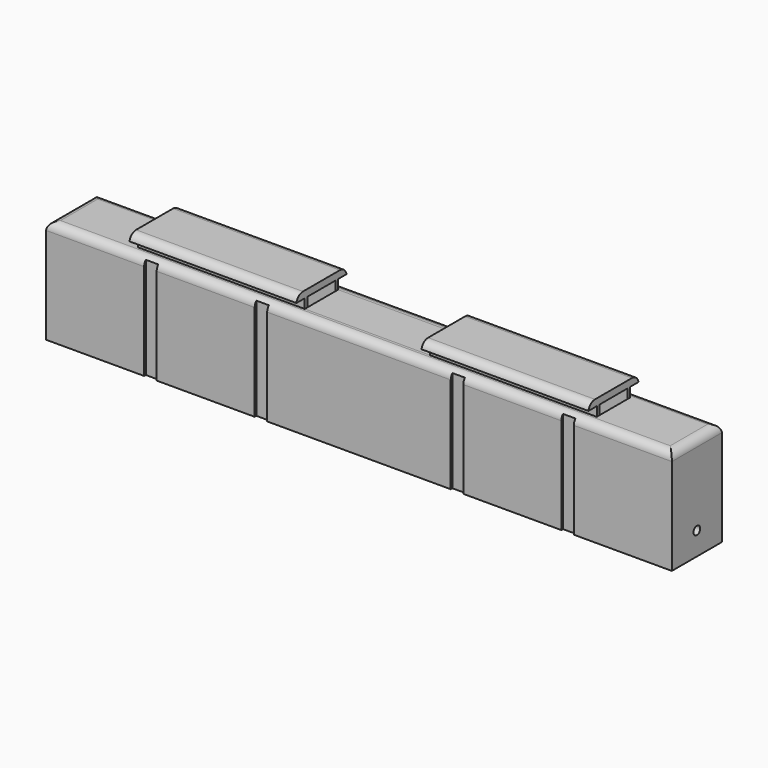
from build123d import *

# Parameters (mm, degrees)
F0_W           = 10.16
F0_H           = 2.54
F1_DEPTH       = 6.35
F2_DEPTH       = 0.635
F4_DEPTH       = 27.94
F6_R           = 0.254
F7_DEPTH       = 38.101
F8_T1_DEPTH    = 6.354829213
F8_T3_DEPTH    = 13.720829213
F10_DEPTH      = 9.652
F11_DEPTH      = 17.272
F12_W          = 2.5144716492
F12_H          = 3.5254987888
F13_DEPTH      = 3.81
F14_DEPTH      = 3.302
F16_DEPTH      = 10.16
F18_DEPTH      = 10.16
F20_DEPTH      = 10.16
F21_T1_DEPTH   = 12.6606557729
F23_DEPTH      = 10.16
F24_T1_DEPTH   = 12.6606557729
F24_2_T1_DEPTH = 8.0250460087
F24_2_T3_DEPTH = 8.0034146065
F24_2_T5_DEPTH = 8.0034146065
F24_2_T7_DEPTH = 8.0250460087
F25_W          = 7.62
F25_H          = 2.54
F26_DEPTH      = 4.5568268582
F27_W          = 7.62
F27_H          = 2.54
F28_DEPTH      = 4.5568268582


# Not quite as in the source:
# - a fillet or chamfer that OpenCascade refuses, or shapes differently, is made with other operations: its cross-section is extruded or revolved along the edge and cut away or added


with BuildPart() as f1:
    # F0 (on Top) → F1 (new body)
    with BuildSketch(Plane.XY):
        Polygon((13.081, -1.905), (19.05, -1.905), (19.05, 1.905), (13.081, 1.905), (13.081, 1.778), (12.319, 1.778), (12.319, 1.905), (6.35, 1.905), (6.35, 1.778), (5.588, 1.778), (5.588, 1.905), (-5.588, 1.905), (-5.588, 1.778), (-6.35, 1.778), (-6.35, 1.905), (-12.319, 1.905), (-12.319, 1.778), (-13.081, 1.778), (-13.081, 1.905), (-19.05, 1.905), (-19.05, -1.905), (-13.081, -1.905), (-13.081, -1.778), (-12.319, -1.778), (-12.319, -1.905), (-6.35, -1.905), (-6.35, -1.778), (-5.588, -1.778), (-5.588, -1.905), (5.588, -1.905), (5.588, -1.778), (6.35, -1.778), (6.35, -1.905), (12.319, -1.905), (12.319, -1.778), (13.081, -1.778), align=None)
        with Locations((-8.89, 0)):
            Rectangle(F0_W, F0_H, mode=Mode.SUBTRACT)
        with Locations((8.89, 0)):
            Rectangle(F0_W, F0_H, mode=Mode.SUBTRACT)
    extrude(amount=F1_DEPTH)

    # F0 (on Top) → F2 (join)
    with BuildSketch(Plane.XY):
        with Locations((-8.89, 0)):
            Rectangle(F0_W, F0_H)
        with Locations((8.89, 0)):
            Rectangle(F0_W, F0_H)
    extrude(amount=F2_DEPTH)

    # F3 (on face) → F4 (cut, through all)
    with BuildSketch(Plane.YZ.offset(-13.97)):
        Polygon((-0.4982374667, 0.381), (0.4982374667, 0.381), (0.4982374667, 0.889), (1.27, 1.397), (1.27, 5.461), (-1.27, 5.461), (-1.27, 1.397), (-0.4982374667, 0.889), align=None)
    extrude(amount=F4_DEPTH, mode=Mode.SUBTRACT)

    # F6 (on face) → F7 (cut, through all)
    with BuildSketch(Plane(origin=(-19.05, 0, 0), x_dir=(0, -1, 0), z_dir=(-1, 0, 0))):
        with Locations((0, 1.397)):
            Circle(F6_R)
    extrude(amount=-F7_DEPTH, mode=Mode.SUBTRACT)

    # F8: fillet of radius 0.508 on 4 edges, made by hand

    # F8_s2 → F8_t1 (cut)
    with BuildSketch(Plane.XZ.offset(-3.1774146065)):
        with BuildLine():
            ThreePointArc((-18.5410343146, 6.3504), (-18.9012102448, 6.2012102448), (-19.0504, 5.8410343146))
            Line((-19.0504, 5.8410343146), (-19.1013365685, 5.8410343146))
            ThreePointArc((-19.1013365685, 5.8410343146), (-19.1009365685, 6.0955171573), (-19.1009365685, 6.35))
            Line((-19.1009365685, 6.35), (-19.05, 6.4009365685))
            ThreePointArc((-19.05, 6.4009365685), (-18.7955171573, 6.4009365685), (-18.5410343146, 6.4013365685))
            Line((-18.5410343146, 6.4013365685), (-18.5410343146, 6.3504))
        make_face()
        with BuildLine():
            ThreePointArc((19.0504, 5.8410343146), (18.9012102448, 6.2012102448), (18.5410343146, 6.3504))
            Line((18.5410343146, 6.3504), (18.5410343146, 6.4013365685))
            ThreePointArc((18.5410343146, 6.4013365685), (18.7955171573, 6.4009365685), (19.05, 6.4009365685))
            Line((19.05, 6.4009365685), (19.1009365685, 6.35))
            ThreePointArc((19.1009365685, 6.35), (19.1009365685, 6.0955171573), (19.1013365685, 5.8410343146))
            Line((19.1013365685, 5.8410343146), (19.0504, 5.8410343146))
        make_face()
    extrude(amount=F8_T1_DEPTH, mode=Mode.SUBTRACT)

    # F8_s4 → F8_t3 (cut)
    with BuildSketch(Plane.YZ.offset(-6.8604146065)):
        with BuildLine():
            ThreePointArc((1.3960343146, 6.3504), (1.7562102448, 6.2012102448), (1.9054, 5.8410343146))
            Line((1.9054, 5.8410343146), (1.9563365685, 5.8410343146))
            ThreePointArc((1.9563365685, 5.8410343146), (1.9559365685, 6.0955171573), (1.9559365685, 6.35))
            Line((1.9559365685, 6.35), (1.905, 6.4009365685))
            ThreePointArc((1.905, 6.4009365685), (1.6505171573, 6.4009365685), (1.3960343146, 6.4013365685))
            Line((1.3960343146, 6.4013365685), (1.3960343146, 6.3504))
        make_face()
        with BuildLine():
            ThreePointArc((-1.3960343146, 6.3504), (-1.7562102448, 6.2012102448), (-1.9054, 5.8410343146))
            Line((-1.9054, 5.8410343146), (-1.9563365685, 5.8410343146))
            ThreePointArc((-1.9563365685, 5.8410343146), (-1.9559365685, 6.0955171573), (-1.9559365685, 6.35))
            Line((-1.9559365685, 6.35), (-1.905, 6.4009365685))
            ThreePointArc((-1.905, 6.4009365685), (-1.6505171573, 6.4009365685), (-1.3960343146, 6.4013365685))
            Line((-1.3960343146, 6.4013365685), (-1.3960343146, 6.3504))
        make_face()
    extrude(amount=F8_T3_DEPTH, mode=Mode.SUBTRACT)


with BuildPart() as f10:
    # F9 (on face) → F10 (new body, through all)
    with BuildSketch(Plane(origin=(-3.81, 0, 0), x_dir=(0, -1, 0), z_dir=(-1, 0, 0))):
        with BuildLine():
            Line((-0.0880359173, 1.4812426976), (-0.381, 5.207))
            ThreePointArc((-0.381, 5.207), (-0.9198153673, 4.9838153673), (-1.143, 4.445))
            Line((-1.143, 4.445), (-1.143, 1.397))
            Line((-1.143, 1.397), (-0.4176268994, 0.8964751032))
            ThreePointArc((-0.4176268994, 0.8964751032), (0, 0.4231398893), (0.4176268994, 0.8964751032))
            Line((0.4176268994, 0.8964751032), (1.143, 1.397))
            Line((1.143, 1.397), (1.143, 4.445))
            ThreePointArc((1.143, 4.445), (0.9198153673, 4.9838153673), (0.381, 5.207))
            Line((0.381, 5.207), (0.0880359173, 1.4812426976))
            ThreePointArc((0.0880359173, 1.4812426976), (0.1267060772, 1.4088201678), (0.0771916931, 1.3433317729))
            Line((0.0771916931, 1.3433317729), (0.0768500527, 1.338986977))
            Line((0.0768500527, 1.338986977), (0.0526172437, 1.0308073381))
            ThreePointArc((0.0526172437, 1.0308073381), (0, 0.6500122176), (-0.0526172437, 1.0308073381))
            Line((-0.0526172437, 1.0308073381), (-0.0768500527, 1.338986977))
            Line((-0.0768500527, 1.338986977), (-0.0771916931, 1.3433317729))
            ThreePointArc((-0.0771916931, 1.3433317729), (-0.1904525618, 1.4038076485), (-0.0880359173, 1.4812426976))
        make_face()
    extrude(amount=F10_DEPTH)

    # F11 (add, through all): a face of the model
    f11_faces = [f10.faces().sort_by_distance(p)[0] for p in [
        (-3.81, 0, 0.5969923029),
    ]]
    extrude(f11_faces, amount=F11_DEPTH)

    # F12 (on Right) → F13 (cut, symmetric)
    with BuildSketch(Plane.YZ):
        with Locations((-0.0007677008, 3.5559225362)):
            Rectangle(F12_W, F12_H)
    extrude(amount=F13_DEPTH, both=True, mode=Mode.SUBTRACT)


with BuildPart() as f14:
    # F14 (new): a face of the model
    f14_faces = [f1.part.faces().sort_by_distance(p)[0] for p in [
        (0, 0, 5.461),
    ]]
    extrude(f14_faces, amount=F14_DEPTH)

    # F27 (on face) → F28 (join, through all)
    with BuildSketch(Plane.XY.offset(1.7931731418)):
        Rectangle(F27_W, F27_H)
    extrude(amount=F28_DEPTH)


with BuildPart() as f1_1:
    add(f1.part)

    # F15 (on face) → F16 (cut, through all)
    with BuildSketch(Plane.YZ.offset(-13.97)):
        with BuildLine():
            Line((1.27, 4.572), (1.27, 4.318))
            ThreePointArc((1.27, 4.318), (1.397, 4.445), (1.27, 4.572))
        make_face()
        with BuildLine():
            ThreePointArc((-1.27, 4.572), (-1.397, 4.445), (-1.27, 4.318))
            Line((-1.27, 4.318), (-1.27, 4.572))
        make_face()
        with BuildLine():
            Line((-1.27, 4.953), (-1.27, 5.207))
            ThreePointArc((-1.27, 5.207), (-1.397, 5.08), (-1.27, 4.953))
        make_face()
        with BuildLine():
            ThreePointArc((1.27, 4.953), (1.397, 5.08), (1.27, 5.207))
            Line((1.27, 5.207), (1.27, 4.953))
        make_face()
    extrude(amount=F16_DEPTH, mode=Mode.SUBTRACT)

    # F17 (on face) → F18 (cut, through all)
    with BuildSketch(Plane(origin=(13.97, 0, 0), x_dir=(0, -1, 0), z_dir=(-1, 0, 0))):
        with BuildLine():
            Line((1.27, 4.5734065802), (1.27, 4.3194065802))
            ThreePointArc((1.27, 4.3194065802), (1.397, 4.4464065802), (1.27, 4.5734065802))
        make_face()
        with BuildLine():
            ThreePointArc((-1.27, 4.5734065802), (-1.397, 4.4464065802), (-1.27, 4.3194065802))
            Line((-1.27, 4.3194065802), (-1.27, 4.5734065802))
        make_face()
        with BuildLine():
            Line((-1.27, 4.9544065802), (-1.27, 5.2084065802))
            ThreePointArc((-1.27, 5.2084065802), (-1.397, 5.0814065802), (-1.27, 4.9544065802))
        make_face()
        with BuildLine():
            ThreePointArc((1.27, 4.9544065802), (1.397, 5.0814065802), (1.27, 5.2084065802))
            Line((1.27, 5.2084065802), (1.27, 4.9544065802))
        make_face()
    extrude(amount=F18_DEPTH, mode=Mode.SUBTRACT)

    # F24#2: fillet of radius 0.508 on 8 edges, made by hand

    # F24_2_s2 → F24_2_t1 (cut)
    with BuildSketch(Plane.YZ.offset(11.8085853935)):
        with BuildLine():
            ThreePointArc((-1.9054, 5.8410343146), (-1.7562102448, 6.2012102448), (-1.3960343146, 6.3504))
            Line((-1.3960343146, 6.3504), (-1.3960343146, 6.4013365685))
            ThreePointArc((-1.3960343146, 6.4013365685), (-1.6505171573, 6.4009365685), (-1.905, 6.4009365685))
            Line((-1.905, 6.4009365685), (-1.9559365685, 6.35))
            ThreePointArc((-1.9559365685, 6.35), (-1.9559365685, 6.0955171573), (-1.9563365685, 5.8410343146))
            Line((-1.9563365685, 5.8410343146), (-1.9054, 5.8410343146))
        make_face()
        with BuildLine():
            ThreePointArc((1.3960343146, 6.3504), (1.7562102448, 6.2012102448), (1.9054, 5.8410343146))
            Line((1.9054, 5.8410343146), (1.9563365685, 5.8410343146))
            ThreePointArc((1.9563365685, 5.8410343146), (1.9559365685, 6.0955171573), (1.9559365685, 6.35))
            Line((1.9559365685, 6.35), (1.905, 6.4009365685))
            ThreePointArc((1.905, 6.4009365685), (1.6505171573, 6.4009365685), (1.3960343146, 6.4013365685))
            Line((1.3960343146, 6.4013365685), (1.3960343146, 6.3504))
        make_face()
    extrude(amount=F24_2_T1_DEPTH, mode=Mode.SUBTRACT)

    # F24_2_s4 → F24_2_t3 (cut)
    with BuildSketch(Plane.YZ.offset(5.588)):
        with BuildLine():
            ThreePointArc((-1.3960343146, 6.3504), (-1.7562102448, 6.2012102448), (-1.9054, 5.8410343146))
            Line((-1.9054, 5.8410343146), (-1.9563365685, 5.8410343146))
            ThreePointArc((-1.9563365685, 5.8410343146), (-1.9559365685, 6.0955171573), (-1.9559365685, 6.35))
            Line((-1.9559365685, 6.35), (-1.905, 6.4009365685))
            ThreePointArc((-1.905, 6.4009365685), (-1.6505171573, 6.4009365685), (-1.3960343146, 6.4013365685))
            Line((-1.3960343146, 6.4013365685), (-1.3960343146, 6.3504))
        make_face()
        with BuildLine():
            ThreePointArc((1.3960343146, 6.3504), (1.7562102448, 6.2012102448), (1.9054, 5.8410343146))
            Line((1.9054, 5.8410343146), (1.9563365685, 5.8410343146))
            ThreePointArc((1.9563365685, 5.8410343146), (1.9559365685, 6.0955171573), (1.9559365685, 6.35))
            Line((1.9559365685, 6.35), (1.905, 6.4009365685))
            ThreePointArc((1.905, 6.4009365685), (1.6505171573, 6.4009365685), (1.3960343146, 6.4013365685))
            Line((1.3960343146, 6.4013365685), (1.3960343146, 6.3504))
        make_face()
    extrude(amount=F24_2_T3_DEPTH, mode=Mode.SUBTRACT)

    # F24_2_s6 → F24_2_t5 (cut)
    with BuildSketch(Plane.YZ.offset(-13.5914146065)):
        with BuildLine():
            ThreePointArc((-1.3960343146, 6.3504), (-1.7562102448, 6.2012102448), (-1.9054, 5.8410343146))
            Line((-1.9054, 5.8410343146), (-1.9563365685, 5.8410343146))
            ThreePointArc((-1.9563365685, 5.8410343146), (-1.9559365685, 6.0955171573), (-1.9559365685, 6.35))
            Line((-1.9559365685, 6.35), (-1.905, 6.4009365685))
            ThreePointArc((-1.905, 6.4009365685), (-1.6505171573, 6.4009365685), (-1.3960343146, 6.4013365685))
            Line((-1.3960343146, 6.4013365685), (-1.3960343146, 6.3504))
        make_face()
        with BuildLine():
            ThreePointArc((1.3960343146, 6.3504), (1.7562102448, 6.2012102448), (1.9054, 5.8410343146))
            Line((1.9054, 5.8410343146), (1.9563365685, 5.8410343146))
            ThreePointArc((1.9563365685, 5.8410343146), (1.9559365685, 6.0955171573), (1.9559365685, 6.35))
            Line((1.9559365685, 6.35), (1.905, 6.4009365685))
            ThreePointArc((1.905, 6.4009365685), (1.6505171573, 6.4009365685), (1.3960343146, 6.4013365685))
            Line((1.3960343146, 6.4013365685), (1.3960343146, 6.3504))
        make_face()
    extrude(amount=F24_2_T5_DEPTH, mode=Mode.SUBTRACT)

    # F24_2_s8 → F24_2_t7 (cut)
    with BuildSketch(Plane.YZ.offset(-19.8336314022)):
        with BuildLine():
            ThreePointArc((-1.3960343146, 6.3504), (-1.7562102448, 6.2012102448), (-1.9054, 5.8410343146))
            Line((-1.9054, 5.8410343146), (-1.9563365685, 5.8410343146))
            ThreePointArc((-1.9563365685, 5.8410343146), (-1.9559365685, 6.0955171573), (-1.9559365685, 6.35))
            Line((-1.9559365685, 6.35), (-1.905, 6.4009365685))
            ThreePointArc((-1.905, 6.4009365685), (-1.6505171573, 6.4009365685), (-1.3960343146, 6.4013365685))
            Line((-1.3960343146, 6.4013365685), (-1.3960343146, 6.3504))
        make_face()
        with BuildLine():
            ThreePointArc((1.3960343146, 6.3504), (1.7562102448, 6.2012102448), (1.9054, 5.8410343146))
            Line((1.9054, 5.8410343146), (1.9563365685, 5.8410343146))
            ThreePointArc((1.9563365685, 5.8410343146), (1.9559365685, 6.0955171573), (1.9559365685, 6.35))
            Line((1.9559365685, 6.35), (1.905, 6.4009365685))
            ThreePointArc((1.905, 6.4009365685), (1.6505171573, 6.4009365685), (1.3960343146, 6.4013365685))
            Line((1.3960343146, 6.4013365685), (1.3960343146, 6.3504))
        make_face()
    extrude(amount=F24_2_T7_DEPTH, mode=Mode.SUBTRACT)

    # F25 (on face) → F26 (cut, through all)
    with BuildSketch(Plane.XY.offset(6.35)):
        Rectangle(F25_W, F25_H)
    extrude(amount=-F26_DEPTH, mode=Mode.SUBTRACT)


with BuildPart() as f20:
    # F19 (on face) → F20 (new body, through all)
    with BuildSketch(Plane(origin=(13.97, 0, 0), x_dir=(0, -1, 0), z_dir=(-1, 0, 0))):
        with BuildLine():
            Line((-1.27, 4.9036065802), (-1.27, 3.7397078704))
            Line((-1.27, 3.7397078704), (-1.0667999741, 3.7397078704))
            Line((-1.0667999741, 3.7397078704), (-1.0667999741, 3.9429078963))
            Line((-1.0667999741, 3.9429078963), (-1.0667999741, 6.9219944999))
            Line((-1.0667999741, 6.9219944999), (1.0667999741, 6.9219944999))
            Line((1.0667999741, 6.9219944999), (1.0667999741, 4.4092186605))
            Line((1.0667999741, 4.4092186605), (1.0667999741, 3.7397078704))
            Line((1.0667999741, 3.7397078704), (1.27, 3.7397078704))
            Line((1.27, 3.7397078704), (1.27, 4.9036065802))
            ThreePointArc((1.27, 4.9036065802), (1.397, 5.0306065802), (1.27, 5.1576065802))
            Line((1.27, 5.1576065802), (1.27, 5.5386065802))
            ThreePointArc((1.27, 5.5386065802), (1.397, 5.6656065802), (1.27, 5.7926065802))
            Line((1.27, 5.7926065802), (1.27, 6.9219944999))
            Line((1.27, 6.9219944999), (1.905, 6.9219944999))
            Line((1.905, 6.9219944999), (1.905, 7.340928074))
            Line((1.905, 7.340928074), (-1.905, 7.340928074))
            Line((-1.905, 7.340928074), (-1.905, 6.9219944999))
            Line((-1.905, 6.9219944999), (-1.27, 6.9219944999))
            Line((-1.27, 6.9219944999), (-1.27, 5.7926065802))
            ThreePointArc((-1.27, 5.7926065802), (-1.397, 5.6656065802), (-1.27, 5.5386065802))
            Line((-1.27, 5.5386065802), (-1.27, 5.1576065802))
            ThreePointArc((-1.27, 5.1576065802), (-1.397, 5.0306065802), (-1.27, 4.9036065802))
        make_face()
    extrude(amount=F20_DEPTH)

    # F21: fillet of radius 0.508 on 2 edges, made by hand

    # F21_s2 → F21_t1 (cut)
    with BuildSketch(Plane.YZ.offset(2.5596721136)):
        with BuildLine():
            ThreePointArc((1.905, 6.9219944999), (1.7310729653, 7.2223569791), (1.4048688454, 7.340928074))
            Line((1.4048688454, 7.340928074), (1.905, 7.340928074))
            Line((1.905, 7.340928074), (1.905, 6.9219944999))
        make_face()
        with BuildLine():
            ThreePointArc((-1.4048688454, 7.340928074), (-1.7310729653, 7.2223569791), (-1.905, 6.9219944999))
            Line((-1.905, 6.9219944999), (-1.905, 7.340928074))
            Line((-1.905, 7.340928074), (-1.4048688454, 7.340928074))
        make_face()
    extrude(amount=F21_T1_DEPTH, mode=Mode.SUBTRACT)


with BuildPart() as f23:
    # F22 (on face) → F23 (new body, through all)
    with BuildSketch(Plane.YZ.offset(-13.97)):
        with BuildLine():
            Line((-1.27, 4.9036112368), (-1.27, 3.739712527))
            Line((-1.27, 3.739712527), (-1.0667999741, 3.739712527))
            Line((-1.0667999741, 3.739712527), (-1.0667999741, 3.942912553))
            Line((-1.0667999741, 3.942912553), (-1.0667999741, 6.9219991565))
            Line((-1.0667999741, 6.9219991565), (1.0667999741, 6.9219991565))
            Line((1.0667999741, 6.9219991565), (1.0667999741, 4.4092233171))
            Line((1.0667999741, 4.4092233171), (1.0667999741, 3.739712527))
            Line((1.0667999741, 3.739712527), (1.27, 3.739712527))
            Line((1.27, 3.739712527), (1.27, 4.9036112368))
            ThreePointArc((1.27, 4.9036112368), (1.397, 5.0306112368), (1.27, 5.1576112368))
            Line((1.27, 5.1576112368), (1.27, 5.5386112368))
            ThreePointArc((1.27, 5.5386112368), (1.397, 5.6656112368), (1.27, 5.7926112368))
            Line((1.27, 5.7926112368), (1.27, 6.9219991565))
            Line((1.27, 6.9219991565), (1.905, 6.9219991565))
            Line((1.905, 6.9219991565), (1.905, 7.3409327306))
            Line((1.905, 7.3409327306), (-1.905, 7.3409327306))
            Line((-1.905, 7.3409327306), (-1.905, 6.9219991565))
            Line((-1.905, 6.9219991565), (-1.27, 6.9219991565))
            Line((-1.27, 6.9219991565), (-1.27, 5.7926112368))
            ThreePointArc((-1.27, 5.7926112368), (-1.397, 5.6656112368), (-1.27, 5.5386112368))
            Line((-1.27, 5.5386112368), (-1.27, 5.1576112368))
            ThreePointArc((-1.27, 5.1576112368), (-1.397, 5.0306112368), (-1.27, 4.9036112368))
        make_face()
    extrude(amount=F23_DEPTH)

    # F24: fillet of radius 0.508 on 2 edges, made by hand

    # F24_s2 → F24_t1 (cut)
    with BuildSketch(Plane.YZ.offset(-15.2203278864)):
        with BuildLine():
            ThreePointArc((-1.905, 6.9219991565), (-1.7310729653, 7.2223616357), (-1.4048688454, 7.3409327306))
            Line((-1.4048688454, 7.3409327306), (-1.905, 7.3409327306))
            Line((-1.905, 7.3409327306), (-1.905, 6.9219991565))
        make_face()
        with BuildLine():
            ThreePointArc((1.4048688454, 7.3409327306), (1.7310729653, 7.2223616357), (1.905, 6.9219991565))
            Line((1.905, 6.9219991565), (1.905, 7.3409327306))
            Line((1.905, 7.3409327306), (1.4048688454, 7.3409327306))
        make_face()
    extrude(amount=F24_T1_DEPTH, mode=Mode.SUBTRACT)


solid = Compound([f10.part, f14.part, f1_1.part, f20.part, f23.part])
